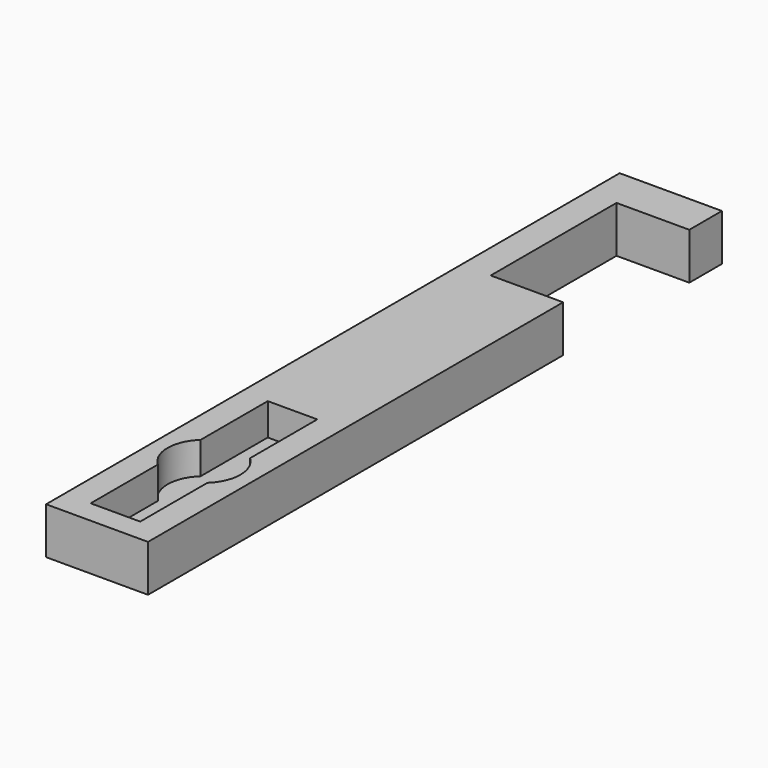
from build123d import *

# Parameters (mm, degrees)
F0_W     = 12.5
F0_H     = 7
F1_DEPTH = 8
F2_DEPTH = 2.5


# Not quite as in the source:
# - a feature names something its author has since deleted; it is built from what else it names


with BuildPart() as f1:
    # F0 (on Top) → F1 (new body)
    with BuildSketch(Plane.XY):
        Polygon((-3.75, 44.5469365077), (-3.6919084378, 44.5469365077), (-3.6919084378, 71.5469365077), (-3.6919084378, 78.5469365077), (-8.75, 78.5469365077), (-8.75, 44.5469365077), align=None)
        Polygon((8.75, -44.5469365077), (8.75, 44.5469365077), (3.75, 44.5469365077), (-3.6919084378, 44.5469365077), (-3.75, 44.5469365077), (-8.75, 44.5469365077), (-8.75, -44.5469365077), align=None)
        with BuildLine():
            Line((-4.25, -2.5992627119), (4.25, -2.5992627119))
            Line((4.25, -2.5992627119), (4.25, -17.016687017))
            ThreePointArc((4.25, -17.016687017), (5.7282196187, -19.0992627119), (6.25, -21.5992627119))
            ThreePointArc((6.25, -21.5992627119), (5.7282196187, -24.0992627119), (4.25, -26.1818384069))
            Line((4.25, -26.1818384069), (4.25, -40.5992627119))
            Line((4.25, -40.5992627119), (-4.25, -40.5992627119))
            Line((-4.25, -40.5992627119), (-4.25, -26.1818384069))
            ThreePointArc((-4.25, -26.1818384069), (-6.25, -21.5992627119), (-4.25, -17.016687017))
            Line((-4.25, -17.016687017), (-4.25, -2.5992627119))
        make_face(mode=Mode.SUBTRACT)
        with Locations((2.5580915622, 75.0469365077)):
            Rectangle(F0_W, F0_H)
    extrude(amount=F1_DEPTH)

    # F0 (on Top) → F2 (join)
    with BuildSketch(Plane.XY):
        with BuildLine():
            Line((4.25, -40.5992627119), (4.25, -26.1818384069))
            ThreePointArc((4.25, -26.1818384069), (0, -27.8492627119), (-4.25, -26.1818384069))
            Line((-4.25, -26.1818384069), (-4.25, -40.5992627119))
            Line((-4.25, -40.5992627119), (4.25, -40.5992627119))
        make_face()
        with BuildLine():
            Line((4.25, -26.1818384069), (4.25, -17.016687017))
            ThreePointArc((4.25, -17.016687017), (0, -15.3492627119), (-4.25, -17.016687017))
            Line((-4.25, -17.016687017), (-4.25, -26.1818384069))
            ThreePointArc((-4.25, -26.1818384069), (0, -27.8492627119), (4.25, -26.1818384069))
        make_face()
        with BuildLine():
            Line((4.25, -17.016687017), (4.25, -2.5992627119))
            Line((4.25, -2.5992627119), (-4.25, -2.5992627119))
            Line((-4.25, -2.5992627119), (-4.25, -17.016687017))
            ThreePointArc((-4.25, -17.016687017), (0, -15.3492627119), (4.25, -17.016687017))
        make_face()
        with BuildLine():
            ThreePointArc((6.25, -21.5992627119), (5.7282196187, -19.0992627119), (4.25, -17.016687017))
            Line((4.25, -17.016687017), (4.25, -26.1818384069))
            ThreePointArc((4.25, -26.1818384069), (5.7282196187, -24.0992627119), (6.25, -21.5992627119))
        make_face()
        with BuildLine():
            Line((-4.25, -26.1818384069), (-4.25, -17.016687017))
            ThreePointArc((-4.25, -17.016687017), (-6.25, -21.5992627119), (-4.25, -26.1818384069))
        make_face()
    extrude(amount=F2_DEPTH)


solid = f1.part
